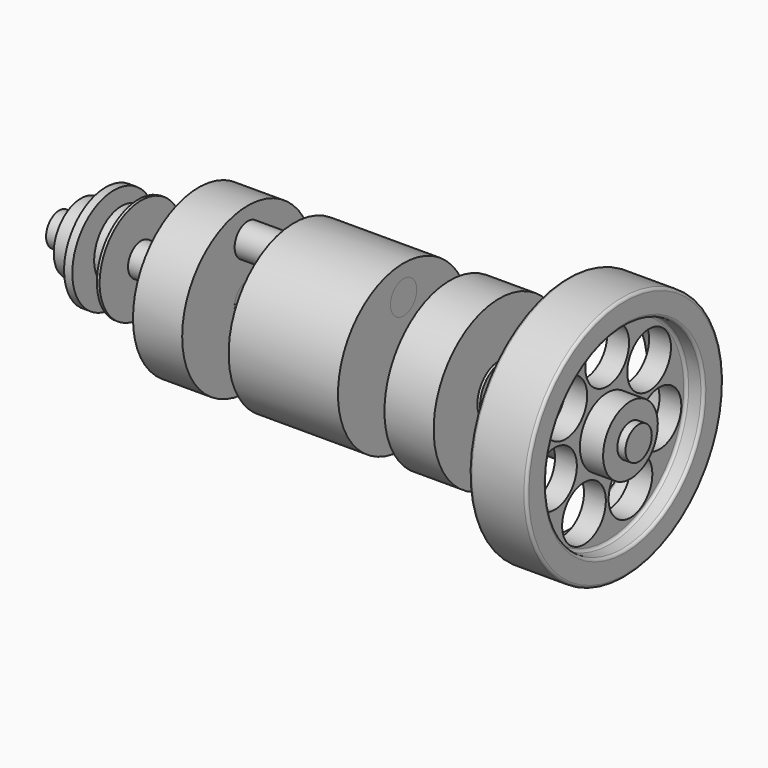
from build123d import *

# Parameters (mm, degrees)
F0_R          = 30
F0_R_2        = 6
F1_DEPTH      = 20
F2_DEPTH      = 55
F2_DEPTH_BACK = 20
F3_DEPTH      = 55
F3_DEPTH_BACK = 20
F4_R          = 30
F4_R_2        = 6
F4_R_3        = 10
F5_DEPTH      = 18
F7_ANGLE      = 180
F8_DEPTH      = 51
F8_DEPTH_BACK = 18
F9_DEPTH      = 1
F13_R         = 10
F14_DEPTH     = 8
F15_R         = 1
F18_R         = 12.5
F18_R_2       = 6
F19_DEPTH     = 12
F18_R_3       = 19
F20_DEPTH     = 3
F21_R         = 12.5
F21_R_2       = 6
F22_DEPTH     = 9
F23_R         = 19
F23_R_2       = 12.5
F23_R_3       = 6
F24_DEPTH     = 1


with BuildPart() as f1:
    # F0 (on Right) → F1 (new body, symmetric)
    with BuildSketch(Plane.YZ):
        Circle(F0_R)
        with Locations((0, -19)):
            Circle(F0_R_2, mode=Mode.SUBTRACT)
        with Locations((0, 19)):
            Circle(F0_R_2, mode=Mode.SUBTRACT)
    extrude(amount=F1_DEPTH, both=True)


with BuildPart() as f2:
    # F0 (on Right) → F2 (new body, two sides)
    with BuildSketch(Plane.YZ) as f2_sk:
        with Locations((0, 19)):
            Circle(F0_R_2)
    extrude(amount=-F2_DEPTH)
    extrude(f2_sk.sketch, amount=F2_DEPTH_BACK)


with BuildPart() as f3:
    # F0 (on Right) → F3 (new body, two sides)
    with BuildSketch(Plane.YZ) as f3_sk:
        with Locations((0, -19)):
            Circle(F0_R_2)
    extrude(amount=F3_DEPTH)
    extrude(f3_sk.sketch, amount=-F3_DEPTH_BACK)


with BuildPart() as f5:
    # F4 (on face) → F5 (new body)
    with BuildSketch(Plane.YZ.offset(55)):
        Circle(F4_R)
        with Locations((0, -19)):
            Circle(F4_R_2, mode=Mode.SUBTRACT)
        Circle(F4_R_3, mode=Mode.SUBTRACT)
        Circle(F4_R_3)
        Circle(F4_R_2, mode=Mode.SUBTRACT)
    extrude(amount=-F5_DEPTH)


with BuildPart() as f6_1:
    # F6: instance of F5
    add(f5.part.mirror(Plane.YZ))


with BuildPart() as f6_1_1:
    # F7: moved
    add(f6_1.part.rotate(Axis((-55, 0, 0), (-1, 0, 0)), F7_ANGLE))


with BuildPart() as f8:
    # F4 (on face) → F8 (new body, two sides)
    with BuildSketch(Plane.YZ.offset(55)) as f8_sk:
        Circle(F4_R_2)
    extrude(amount=F8_DEPTH)
    extrude(f8_sk.sketch, amount=-F8_DEPTH_BACK)


with BuildPart() as f9:
    # F4 (on face) → F9 (new body)
    with BuildSketch(Plane.YZ.offset(55)):
        Circle(F4_R_3)
        Circle(F4_R_2, mode=Mode.SUBTRACT)
    extrude(amount=F9_DEPTH)


with BuildPart() as f10_1:
    # F10: instance of F8
    add(f8.part.mirror(Plane.YZ))


with BuildPart() as f10_2:
    # F10: instance of F9
    add(f9.part.mirror(Plane.YZ))


with BuildPart() as f12:
    # F11 (on Front) → F12 (revolve)
    with BuildSketch(Plane.XZ):
        Polygon((103, -6), (78, -6), (78, -12.5), (86.5, -12.5), (86.5, -36), (80, -36), (80, -45), (101, -45), (101, -36), (94.5, -36), (94.5, -12.5), (103, -12.5), align=None)
    revolve(axis=Axis((68.9849918365, 0, 0), (1, 0, 0)))

    # F13 (on face) → F14 (cut, through all)
    with BuildSketch(Plane.YZ.offset(94.5)):
        with Locations((-10.6301516084, -22.0737372636)):
            Circle(F13_R)
        with Locations((10.6301516084, -22.0737372636)):
            Circle(F13_R)
        with Locations((23.8857338485, -5.4517628819)):
            Circle(F13_R)
        with Locations((19.1548713205, 15.2755001455)):
            Circle(F13_R)
        with Locations((0, 24.5)):
            Circle(F13_R)
        with Locations((-19.1548713205, 15.2755001455)):
            Circle(F13_R)
        with Locations((-23.8857338485, -5.4517628819)):
            Circle(F13_R)
    extrude(amount=-F14_DEPTH, mode=Mode.SUBTRACT)

    # F15
    f15_edges = [f12.edges().sort_by_distance(p)[0] for p in [
        (101, 0, 45),
        (101, 0, 36),
        (80, 0, 45),
        (80, 0, 36),
        (94.5, 0, 36),
        (86.5, 0, 36),
    ]]
    fillet(f15_edges, radius=F15_R)


with BuildPart() as f16_1:
    # F16: copy of F9
    add(f9.part.moved(Location((21, 0, 0))))


with BuildPart() as f19:
    # F18 (on offset) → F19 (new body)
    with BuildSketch(Plane.YZ.offset(-86)):
        Circle(F18_R)
        Circle(F18_R_2, mode=Mode.SUBTRACT)
    extrude(amount=-F19_DEPTH)

    # F18 (on offset) → F20 (join)
    with BuildSketch(Plane.YZ.offset(-86)):
        Circle(F18_R_3)
        Circle(F18_R, mode=Mode.SUBTRACT)
        Circle(F18_R)
        Circle(F18_R_2, mode=Mode.SUBTRACT)
    extrude(amount=-F20_DEPTH)

    # F21 (on face) → F22 (join)
    with BuildSketch(Plane.YZ.offset(-86)):
        with Locations((3.5, 0)):
            Circle(F21_R)
        Circle(F21_R_2, mode=Mode.SUBTRACT)
    extrude(amount=F22_DEPTH)


with BuildPart() as f24:
    # F23 (on face) → F24 (new body)
    with BuildSketch(Plane.YZ.offset(-77)):
        Circle(F23_R)
        with Locations((3.5, 0)):
            Circle(F23_R_2, mode=Mode.SUBTRACT)
        with Locations((3.5, 0)):
            Circle(F23_R_2)
        Circle(F23_R_3, mode=Mode.SUBTRACT)
    extrude(amount=F24_DEPTH)


solid = Compound([f1.part, f2.part, f3.part, f5.part, f6_1_1.part, f8.part, f9.part, f10_1.part, f10_2.part, f12.part, f16_1.part, f19.part, f24.part])
